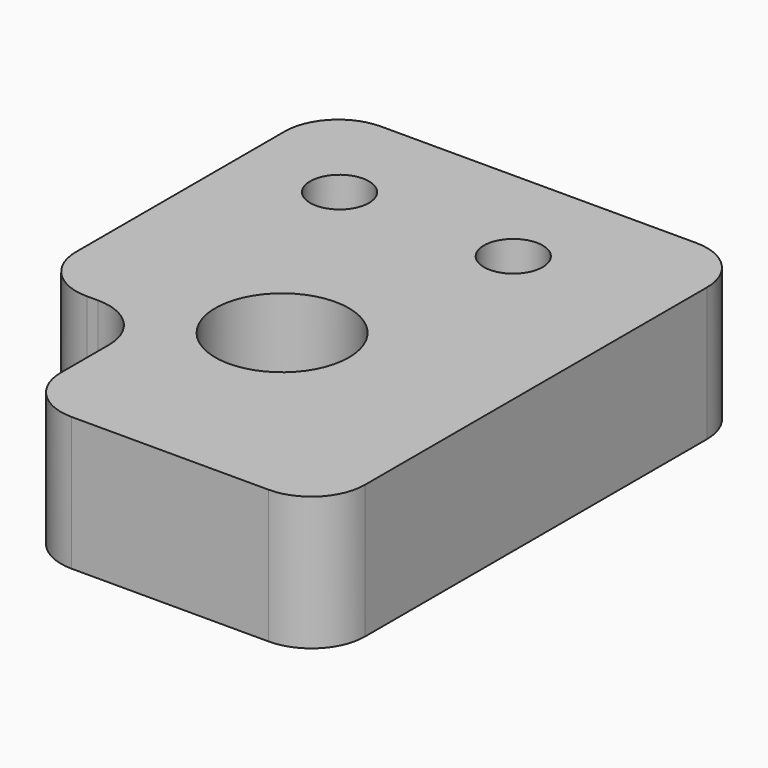
from build123d import *

# Parameters (mm, degrees)
F0_R     = 2.5
F0_R_2   = 1.1
F1_DEPTH = 5
F2_R     = 2


with BuildPart() as f1:
    # F0 (on Top) → F1 (new body)
    with BuildSketch(Plane.XY):
        Polygon((7.9, 8.3929710358), (0, 8.3929710358), (-7.9, 8.3929710358), (-7.9, -5.3654396906), (-3.4737212118, -5.3654396906), (-3.4737212118, -11.6070289642), (0, -11.6070289642), (7.9, -11.6070289642), align=None)
        with Locations((0, -3.6070289642)):
            Circle(F0_R, mode=Mode.SUBTRACT)
        with Locations((-4.25, 4.3929710358)):
            Circle(F0_R_2, mode=Mode.SUBTRACT)
        with Locations((2.25, 4.3929710358)):
            Circle(F0_R_2, mode=Mode.SUBTRACT)
    extrude(amount=F1_DEPTH)

    # F2
    f2_edges = [f1.edges().sort_by_distance(p)[0] for p in [
        (7.9, -11.607029, 2.5),
        (7.9, 8.392971, 2.5),
        (-3.473721, -11.607029, 2.5),
        (-7.9, 8.392971, 2.5),
        (-7.9, -5.36544, 2.5),
        (-3.473721, -5.36544, 2.5),
    ]]
    fillet(f2_edges, radius=F2_R)


solid = f1.part
